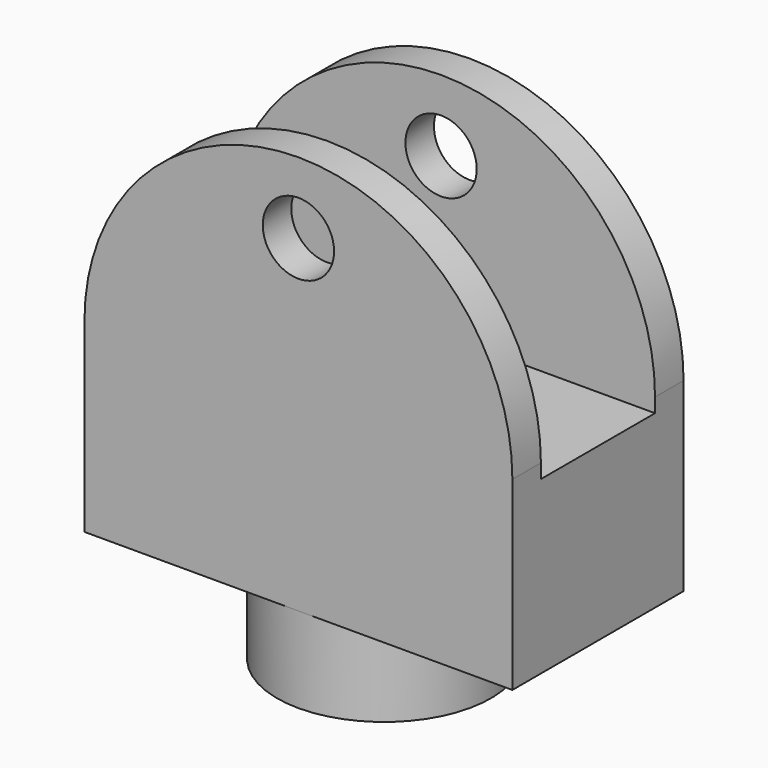
from build123d import *

# Parameters (mm, degrees)
F0_W      = 30
F0_H      = 12
F1_DEPTH  = 15
F2_W      = 30
F2_H      = 1
F3_DEPTH  = 2.5
F4_W      = 30
F4_H      = 1
F5_DEPTH  = 2.5
F6_R      = 2.5
F7_DEPTH  = 15.001
F9_DEPTH  = 6
F10_R     = 6.5
F11_DEPTH = 2


# Not quite as in the source:
# - a feature names something its author has since deleted; it is built from what else it names


with BuildPart() as f1:
    # F0 (on Front) → F1 (new body)
    with BuildSketch(Plane.XZ):
        Rectangle(F0_W, F0_H)
    extrude(amount=F1_DEPTH)

    # F2 (on face) → F3 (join)
    with BuildSketch(Plane(origin=(0, 0, 0), x_dir=(-1, 0, 0), z_dir=(0, 1, 0))):
        with Locations((0, 6.5)):
            Rectangle(F2_W, F2_H)
        with BuildLine():
            ThreePointArc((15, 7), (0, 22), (-15, 7))
            Line((-15, 7), (15, 7))
        make_face()
    extrude(amount=-F3_DEPTH)

    # F4 (on face) → F5 (join)
    with BuildSketch(Plane.XZ.offset(15)):
        with Locations((0, 6.5)):
            Rectangle(F4_W, F4_H)
        with BuildLine():
            ThreePointArc((15, 7), (0, 22), (-15, 7))
            Line((-15, 7), (15, 7))
        make_face()
    extrude(amount=-F5_DEPTH)

    # F6 (on face) → F7 (cut, through all)
    with BuildSketch(Plane.XZ.offset(15)):
        with Locations((-1.01e-08, 17)):
            Circle(F6_R)
    extrude(amount=-F7_DEPTH, mode=Mode.SUBTRACT)

    # F8 (on face) → F9 (join)
    with BuildSketch(Plane(origin=(0, 0, -6), x_dir=(1, 0, 0), z_dir=(0, 0, -1))):
        with BuildLine():
            ThreePointArc((0, 0), (5.3033008589, 2.1966991411), (7.5, 7.5))
            ThreePointArc((7.5, 7.5), (5.3033008589, 12.8033008589), (0, 15))
            ThreePointArc((0, 15), (-7.5, 7.5), (0, 0))
        make_face()
    extrude(amount=F9_DEPTH)

    # F10 (on face) → F11 (cut)
    with BuildSketch(Plane(origin=(0, 0, -12), x_dir=(1, 0, 0), z_dir=(0, 0, -1))):
        with Locations((0, 7.5)):
            Circle(F10_R)
    extrude(amount=-F11_DEPTH, mode=Mode.SUBTRACT)


solid = f1.part
